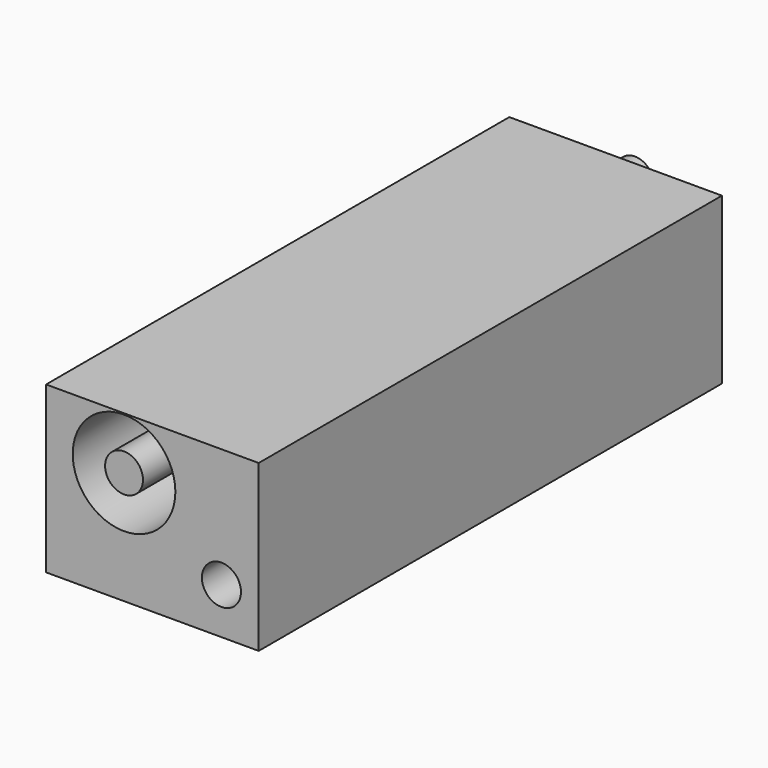
from build123d import *

# Parameters (mm, degrees)
F0_W     = 65.2924329042
F0_H     = 50.8008524776
F0_W_2   = 20.2902685851
F0_H_2   = 12.3683428392
F1_DEPTH = 177.8
F2_R     = 5.8184975352
F3_DEPTH = 177.801
F2_R_2   = 15.7606877534
F2_R_3   = 6.0021596397
F4_DEPTH = 196.114718


# Not quite as in the source:
# - a pattern or mirror of a feature is missing from the dataset's text; its kind, count and spacing are read off the source's solid


with BuildPart() as f1:
    # F0 (on Front) → F1 (new body)
    with BuildSketch(Plane.XZ):
        Rectangle(F0_W, F0_H)
        Rectangle(F0_W_2, F0_H_2, mode=Mode.SUBTRACT)
        Rectangle(F0_W_2, F0_H_2)
    extrude(amount=F1_DEPTH)

    # F2 (on face) → F4 (cut, through all)
    with BuildSketch(Plane.XZ.offset(177.8)):
        with Locations((-8.707053028, 9.2738447711)):
            Circle(F2_R_2)
        with Locations((-8.707053028, 9.2738447711)):
            Circle(F2_R, mode=Mode.SUBTRACT)
        with Locations((21.2008059025, -11.2456455827)):
            Circle(F2_R_3)
    extrude(amount=-F4_DEPTH, mode=Mode.SUBTRACT)


with BuildPart() as f3:
    # F2 (on face) → F3 (new body, through all)
    with BuildSketch(Plane.XZ.offset(177.8)):
        with Locations((-8.707053028, 9.2738447711)):
            Circle(F2_R)
    extrude(amount=-F3_DEPTH)

    # F3_copies: F3 across plane


with BuildPart() as f3_1:
    add(f3.part)
    add(f3.part.mirror(Plane.ZX.offset(-79.743141)))


solid = Compound([f1.part, f3_1.part])
